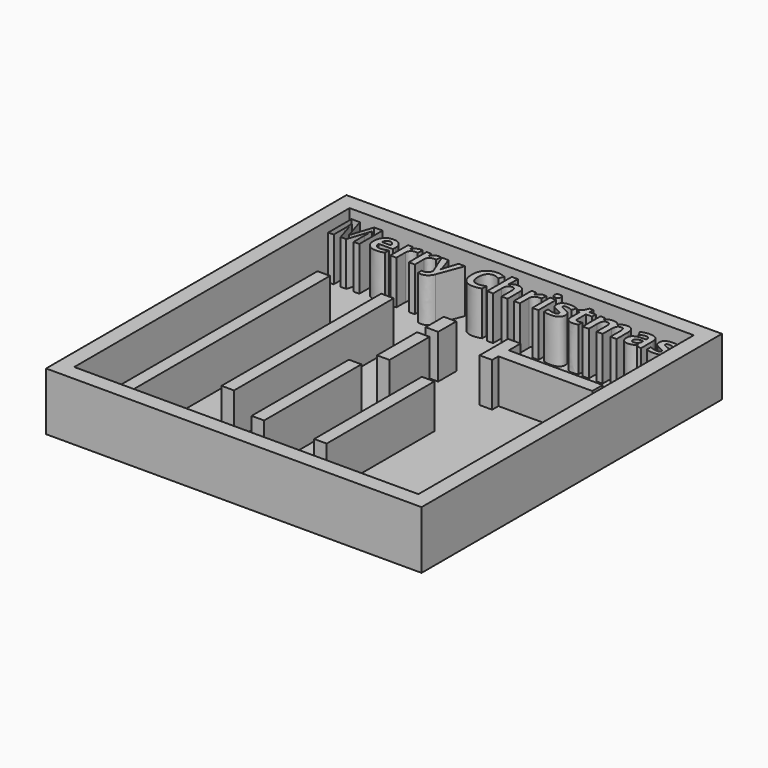
from build123d import *

# Parameters (mm, degrees)
F0_W         = 38.1
F0_H         = 38.1
F1_DEPTH     = 0.79375
F2_W         = 38.1
F2_H         = 38.1
F2_W_2       = 34.925
F2_H_2       = 34.925
F4_DEPTH     = 5.08
F3_W         = 1.27
F3_H         = 25.8311466354
F3_H_2       = 20.2500452605
F3_H_3       = 5.08
F3_H_4       = 2.2981877132
F3_W_2       = 9.525
F3_H_5       = 1.3154447079
F3_H_6       = 13.6612385977
F3_TEXT_SIZE = 4.1358909886
F5_DEPTH     = 4.445
F7_R         = 1.27
F8_DEPTH     = 0.396875
F9_R         = 1.27
F10_DEPTH    = 0.396875


# Not quite as in the source:
# - Text() gives the source's letters only with a copy of the font that has no kerning and outlines rounded to 1/6400 em; it was checked with that copy


with BuildPart() as f1:
    # F0 (on Top) → F1 (new body)
    with BuildSketch(Plane.XY):
        with Locations((0.4642736167, -2.0311219174)):
            Rectangle(F0_W, F0_H)
    extrude(amount=F1_DEPTH)

    # F2 (on face) → F4 (join)
    with BuildSketch(Plane.XY.offset(0.79375)):
        with Locations((0.4642736167, -2.0311219174)):
            Rectangle(F2_W, F2_H)
        with Locations((0.4642736167, -2.0311219174)):
            Rectangle(F2_W_2, F2_H_2, mode=Mode.SUBTRACT)
    extrude(amount=F4_DEPTH)

    # F3 (on face) → F5 (join)
    with BuildSketch(Plane.XY.offset(0.79375)):
        with Locations((-12.3462450465, -6.5780485997)):
            Rectangle(F3_W, F3_H)
        with Locations((-5.9962450465, -3.6410591565)):
            Rectangle(F3_W, F3_H_2)
        Polygon((-1.5512450465, -10.1338352542), (-1.5512450465, -16.3060817868), (-0.2812450465, -16.3060817868), (-0.2812450465, -3.9615887217), (-1.5512450465, -3.9615887217), align=None)
        with Locations((0.3537549535, 0.5535296937)):
            Rectangle(F3_W, F3_H_3)
        with Locations((0.3537549535, 5.3348696171)):
            Rectangle(F3_W, F3_H_4)
        Polygon((7.3387549535, 5.2038254216), (7.3387549535, 6.6996763291), (6.0687549535, 6.6996763291), (6.0687549535, 3.0935296937), (7.3387549535, 3.0935296937), (7.3387549535, 3.8883807138), align=None)
        with Locations((12.1012549535, 4.5461030677)):
            Rectangle(F3_W_2, F3_H_5)
        with Locations((5.4337549535, -9.4754624879)):
            Rectangle(F3_W, F3_H_6)
        with Locations((-16.8340904431, 12.0545337655)):
            Text('Merry Christmas', F3_TEXT_SIZE, font='Open Sans', font_style=FontStyle.BOLD, text_align=(TextAlign.LEFT, TextAlign.BOTTOM))
    extrude(amount=F5_DEPTH)

    # F7 (on face) → F8 (cut)
    with BuildSketch(Plane.XY.offset(0.79375)):
        with Locations((-14.4526879303, -16.8742034584)):
            Circle(F7_R)
    extrude(amount=-F8_DEPTH, mode=Mode.SUBTRACT)

    # F9 (on face) → F10 (cut)
    with BuildSketch(Plane.XY.offset(0.79375)):
        with Locations((13.9287004397, 8.527331174)):
            Circle(F9_R)
    extrude(amount=-F10_DEPTH, mode=Mode.SUBTRACT)


solid = f1.part
